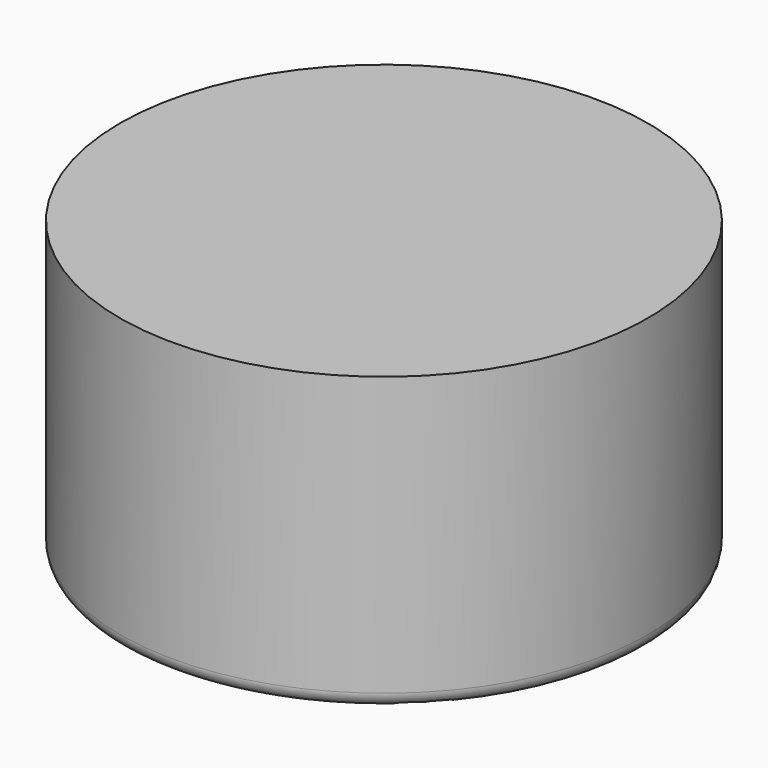
from build123d import *

# Parameters (mm, degrees)
F2_R = 0.5
F3_R = 0.99999


# Not quite as in the source:
# - a fillet or chamfer is up to 0.001 mm smaller than in the source, because OpenCascade refuses the exact size


with BuildPart() as f1:
    # F0 (on Front) → F1 (revolve)
    with BuildSketch(Plane.XZ):
        Polygon((-8.899047263, -1.4357442181), (-8.899047263, -21.4357442181), (-6.899047263, -21.4357442181), (-6.899047263, -3.4357442181), (9.100952737, -3.4357442181), (9.100952737, -1.4357442181), align=None)
    revolve(axis=Axis((9.100952737, 0, -2.4357442181), (0, 0, -1)))

    # F2
    f2_edges = [f1.edges().sort_by_distance(p)[0] for p in [
        (25.100953, 0, -3.435744),
    ]]
    fillet(f2_edges, radius=F2_R)

    # F3 (radius 1 in the source; OpenCascade refuses exactly that, so slightly less here)
    f3_edges = [f1.edges().sort_by_distance(p)[0] for p in [
        (27.100953, 0, -21.435744),
        (25.100953, 0, -21.435744),
    ]]
    fillet(f3_edges, radius=F3_R)


solid = f1.part
